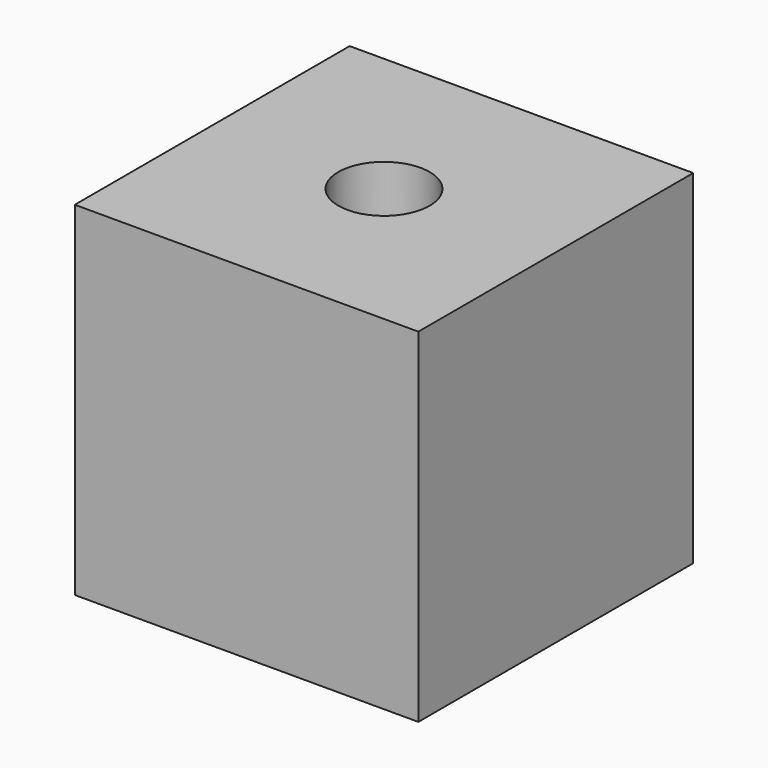
from build123d import *

# Parameters (mm, degrees)
F0_W         = 25.4
F0_H         = 25.4
F1_DEPTH     = 12.7
F3_D         = 6.7564
F3_DEPTH     = 3.81
F3_TIP       = 2.0298273432
F4_TEXT_SIZE = 15.4482433572
F5_DEPTH     = 2


# Not quite as in the source:
# - Text() gives the source's letters only with a copy of the font that has no kerning and outlines rounded to 1/6400 em; it was checked with that copy


with BuildPart() as f1:
    # F0 (on Front) → F1 (new body, symmetric)
    with BuildSketch(Plane.XZ):
        Rectangle(F0_W, F0_H)
    extrude(amount=F1_DEPTH, both=True)

    # F3
    with Locations(Plane.XY.offset(12.7)):
        with Locations((0, 0)):
            Hole(F3_D / 2, depth=F3_DEPTH)
            with Locations((0, 0, -(F3_DEPTH + F3_TIP / 2))):  # 118° drill point
                Cone(0, F3_D / 2, F3_TIP, mode=Mode.SUBTRACT)

    # F4 (on face) → F5 (join)
    with BuildSketch(Plane(origin=(0, 12.7, 0), x_dir=(-1, 0, 0), z_dir=(0, 1, 0))):
        with Locations((-10.3896679357, -4.8911687918)):
            Text('Ari', F4_TEXT_SIZE, font='Open Sans', text_align=(TextAlign.LEFT, TextAlign.BOTTOM))
    extrude(amount=F5_DEPTH)


solid = f1.part
